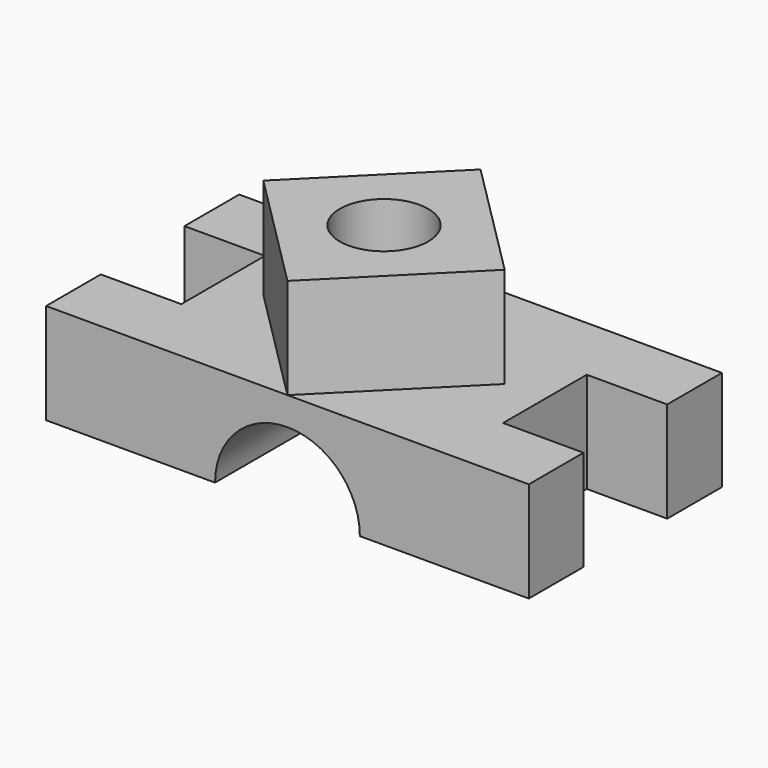
from build123d import *

# Parameters (mm, degrees)
F0_W     = 1200
F0_H     = 600
F1_DEPTH = 250
F2_W     = 400
F2_H     = 260
F3_DEPTH = 250.001
F5_DEPTH = 600.001
F7_DEPTH = 250
F8_R     = 110
F9_DEPTH = 500.001


# Not quite as in the source:
# - a feature names something its author has since deleted; it is built from what else it names


with BuildPart() as f1:
    # F0 (on Top) → F1 (new body)
    with BuildSketch(Plane.XY):
        Rectangle(F0_W, F0_H)
    extrude(amount=F1_DEPTH)

    # F2 (on face) → F3 (cut, through all)
    with BuildSketch(Plane.XY.offset(250)):
        with Locations((-600, 0)):
            Rectangle(F2_W, F2_H)
        with Locations((600, 0)):
            Rectangle(F2_W, F2_H)
    extrude(amount=-F3_DEPTH, mode=Mode.SUBTRACT)

    # F4 (on face) → F5 (cut, through all)
    with BuildSketch(Plane.XZ.offset(300)):
        with BuildLine():
            Line((-180, 0), (180, 0))
            ThreePointArc((180, 0), (0, 180), (-180, 0))
        make_face()
    extrude(amount=-F5_DEPTH, mode=Mode.SUBTRACT)

    # F6 (on face) → F7 (join)
    with BuildSketch(Plane.XY.offset(250)):
        Polygon((299.9999760684, 0), (0, 300), (-300.0000239316, 0), (0, -300), align=None)
    extrude(amount=F7_DEPTH)

    # F8 (on face) → F9 (cut, through all)
    with BuildSketch(Plane.XY.offset(500)):
        Circle(F8_R)
    extrude(amount=-F9_DEPTH, mode=Mode.SUBTRACT)


solid = f1.part
